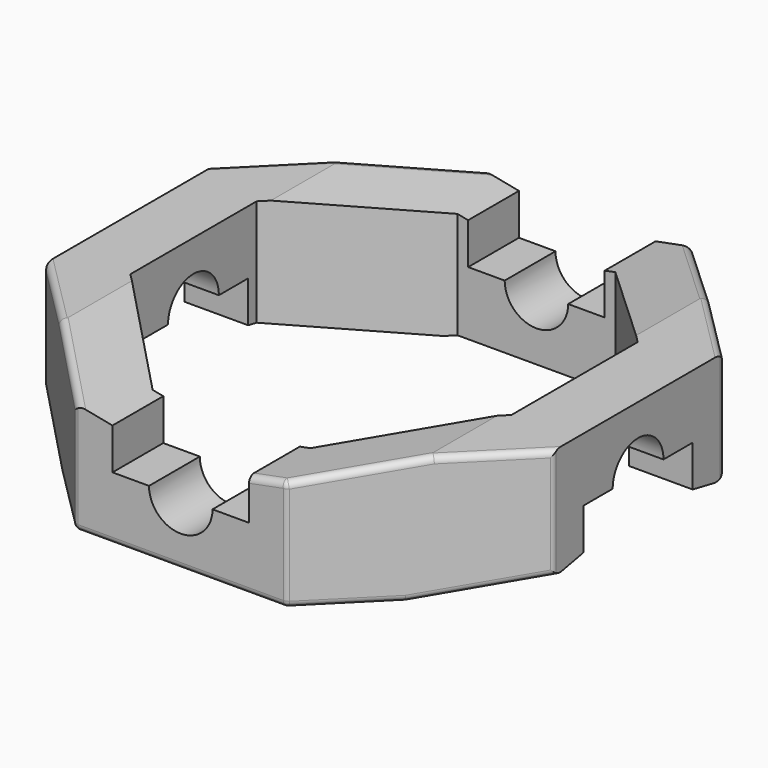
from build123d import *

# Parameters (mm, degrees)
F1_DEPTH      = 40
F2_R          = 10
F3_DEPTH      = 180
F3_DEPTH_BACK = 20
F4_R          = 10
F5_DEPTH      = 20
F5_DEPTH_BACK = 180
F7_DEPTH      = 181.4
F9_DEPTH      = 244.2
F11_DEPTH     = 10
F12_R         = 2
F13_R         = 2


# Not quite as in the source:
# - a feature names something its author has since deleted; it is built from what else it names


with BuildPart() as f1:
    # F0 (on Top) → F1 (new body)
    with BuildSketch(Plane.XY):
        Polygon((-33.1370849898, -80), (33.1370849898, -80), (80, -33.1370849898), (80, 33.1370849898), (33.1370849898, 80), (-33.1370849898, 80), (-80, 33.1370849898), (-80, -33.1370849898), align=None)
        Polygon((60, -24.8528137424), (24.8528137424, -60), (-24.8528137424, -60), (-60, -24.8528137424), (-60, 24.8528137424), (-24.8528137424, 60), (24.8528137424, 60), (60, 24.8528137424), align=None, mode=Mode.SUBTRACT)
    extrude(amount=F1_DEPTH)

    # F2 (on face) → F3 (cut, two sides)
    with BuildSketch(Plane.XZ.offset(80)) as f3_sk:
        with Locations((0, 20)):
            Circle(F2_R)
    extrude(amount=-F3_DEPTH, mode=Mode.SUBTRACT)
    extrude(f3_sk.sketch, amount=F3_DEPTH_BACK, mode=Mode.SUBTRACT)

    # F4 (on face) → F5 (cut, two sides)
    with BuildSketch(Plane.YZ.offset(80)) as f5_sk:
        with Locations((0, 20)):
            Circle(F4_R)
    extrude(amount=F5_DEPTH, mode=Mode.SUBTRACT)
    extrude(f5_sk.sketch, amount=-F5_DEPTH_BACK, mode=Mode.SUBTRACT)

    # F6 (on face) → F7 (cut)
    with BuildSketch(Plane.XZ.offset(80)):
        Polygon((-33.1370849898, 40), (0, 40), (0, 51.6958795488), (-57.5, 51.6958795488), (-71.9271823764, 52.9654417948), (-71.9271823764, 40), (-57.5, 40), (-33.1370849898, 35.2627665258), align=None)
        with BuildLine():
            Line((0, 40), (0, 30))
            ThreePointArc((0, 30), (7.0710678119, 27.0710678119), (10, 20))
            Line((10, 20), (21.5, 20))
            Line((21.5, 20), (21.5, 33))
            Line((21.5, 33), (33.1370849898, 35.2627665258))
            Line((33.1370849898, 35.2627665258), (33.1370849898, 40))
            Line((33.1370849898, 40), (0, 40))
        make_face()
        Polygon((0, 51.6958795488), (0, 40), (33.1370849898, 40), (33.1370849898, 35.2627665258), (57.5, 40), (71.9271823764, 40), (71.9271823764, 52.9654417948), (57.5, 51.6958795488), align=None)
        with BuildLine():
            Line((-21.5, 20), (-10, 20))
            ThreePointArc((-10, 20), (-7.0710678119, 27.0710678119), (0, 30))
            Line((0, 30), (0, 40))
            Line((0, 40), (-33.1370849898, 40))
            Line((-33.1370849898, 40), (-33.1370849898, 35.2627665258))
            Line((-33.1370849898, 35.2627665258), (-21.5, 33))
            Line((-21.5, 33), (-21.5, 20))
        make_face()
    extrude(amount=-F7_DEPTH, mode=Mode.SUBTRACT)

    # F8 (on face) → F9 (cut)
    with BuildSketch(Plane.YZ.offset(80)):
        Polygon((33.1370849898, 0), (0, 0), (0, -11.1064584926), (57.5, -11.1064584926), (66.6687613726, -11.8878306821), (66.6687613726, 0), (57.5, 0), (33.1370849898, 4.7372334742), align=None)
        with BuildLine():
            ThreePointArc((10, 20), (7.0710678119, 12.9289321881), (0, 10))
            Line((0, 10), (0, 0))
            Line((0, 0), (33.1370849898, 0))
            Line((33.1370849898, 0), (33.1370849898, 4.7372334742))
            Line((33.1370849898, 4.7372334742), (21.5, 7))
            Line((21.5, 7), (21.5, 20))
            Line((21.5, 20), (10, 20))
        make_face()
        with BuildLine():
            ThreePointArc((0, 10), (-7.0710678119, 12.9289321881), (-10, 20))
            Line((-10, 20), (-21.5, 20))
            Line((-21.5, 20), (-21.5, 7))
            Line((-21.5, 7), (-33.1370849898, 4.7372334742))
            Line((-33.1370849898, 4.7372334742), (-33.1370849898, 0))
            Line((-33.1370849898, 0), (0, 0))
            Line((0, 0), (0, 10))
        make_face()
        Polygon((0, -11.1064584926), (0, 0), (-33.1370849898, 0), (-33.1370849898, 4.7372334742), (-57.5, 0), (-66.6687613726, 0), (-66.6687613726, -11.8878306821), (-57.5, -11.1064584926), align=None)
    extrude(amount=-F9_DEPTH, mode=Mode.SUBTRACT)

    # F10 (on face) → F11 (cut)
    with BuildSketch(Plane(origin=(56.5685424949, 56.5685424949, 0), x_dir=(-0.7071067812, 0.7071067812, 0), z_dir=(0.7071067812, 0.7071067812, 0))):
        with BuildLine():
            Line((-19.68193107, 12.9813232565), (1.7303785257, 10.0372808895))
            ThreePointArc((1.7303785257, 10.0372808895), (2.0021645777, 10.0093311061), (2.2752246058, 10))
            Line((2.2752246058, 10), (19.1370849898, 10))
            ThreePointArc((19.1370849898, 10), (21.9655121146, 11.1715728753), (23.1370849898, 14))
            Line((23.1370849898, 14), (23.1370849898, 23.055957633))
            ThreePointArc((23.1370849898, 23.055957633), (22.1519966238, 25.6847040718), (19.68193107, 27.0186767435))
            Line((19.68193107, 27.0186767435), (-1.7303785257, 29.9627191105))
            ThreePointArc((-1.7303785257, 29.9627191105), (-2.0021645777, 29.9906688939), (-2.2752246058, 30))
            Line((-2.2752246058, 30), (-19.1370849898, 30))
            ThreePointArc((-19.1370849898, 30), (-21.9655121146, 28.8284271247), (-23.1370849898, 26))
            Line((-23.1370849898, 26), (-23.1370849898, 16.944042367))
            ThreePointArc((-23.1370849898, 16.944042367), (-22.1519966238, 14.3152959282), (-19.68193107, 12.9813232565))
        make_face()
    extrude(amount=-F11_DEPTH, mode=Mode.SUBTRACT)

    # F12
    f12_edges = [f1.edges().sort_by_distance(p)[0] for p in [
        (33.137085, 65.857864, 18.527979),
        (33.965512, 65.029437, 11.171573),
        (41.92708, 57.067869, 10),
    ]]
    fillet(f12_edges, radius=F12_R)

    # F13
    f13_edges = [f1.edges().sort_by_distance(p)[0] for p in [
        (44.387085, 68.75, 0),
        (67.818542, 45.318542, 2.368617),
        (33.137085, 80, 17.631383),
        (45.318542, 67.818542, 37.631383),
        (80, 33.137085, 22.368617),
        (68.75, 44.387085, 40),
        (72.100505, 41.03658, 28.828427),
        (64.138937, 48.998148, 30),
        (57.984287, 55.152798, 29.990669),
        (50.22171, 62.915375, 28.490698),
        (40.904715, 72.23237, 25.684704),
        (40.208153, 72.928932, 18.527979),
        (41.03658, 72.100505, 11.171573),
        (48.998148, 64.138937, 10),
        (55.152798, 57.984287, 10.009331),
        (62.915375, 50.22171, 11.509302),
        (72.23237, 40.904715, 14.315296),
        (72.928932, 40.208153, 21.472021),
        (44.387085, -68.75, 0),
        (33.137085, -80, 17.631383),
        (45.318542, -67.818542, 37.631383),
        (68.75, -44.387085, 40),
        (80, -33.137085, 22.368617),
        (67.818542, -45.318542, 2.368617),
        (0, -80, 0),
        (27.318542, -80, 34.131383),
        (-44.387085, -68.75, 0),
        (-67.818542, -45.318542, 2.368617),
        (-80, -33.137085, 22.368617),
        (-68.75, -44.387085, 40),
        (-45.318542, -67.818542, 37.631383),
        (-33.137085, -80, 17.631383),
        (-44.387085, 68.75, 0),
        (-33.137085, 80, 17.631383),
        (-45.318542, 67.818542, 37.631383),
        (-68.75, 44.387085, 40),
        (-80, 33.137085, 22.368617),
        (-67.818542, 45.318542, 2.368617),
    ]]
    fillet(f13_edges, radius=F13_R)


solid = f1.part
